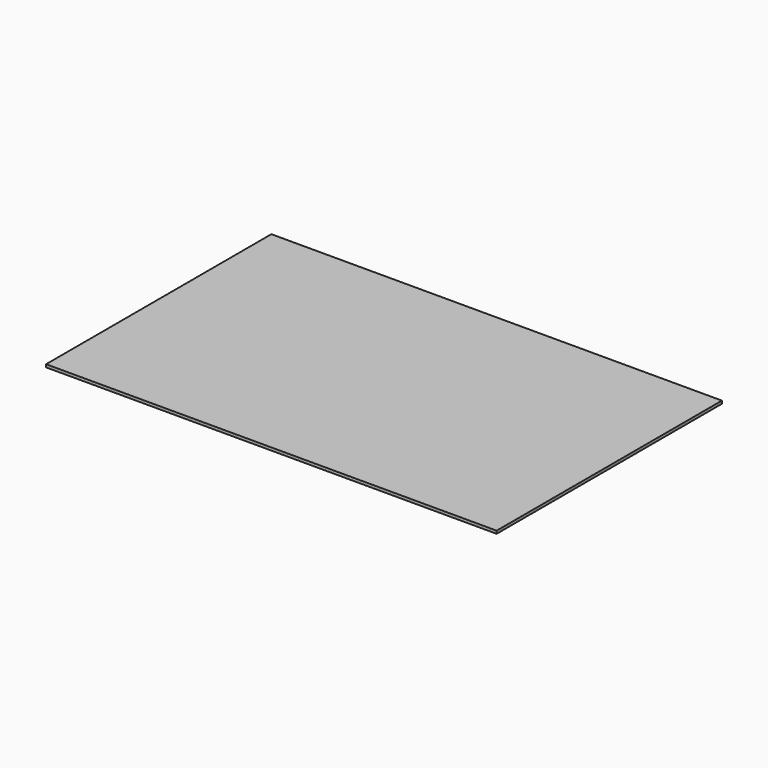
from build123d import *

# Parameters (mm, degrees)
F0_W     = 24384
F0_H     = 15240
F1_DEPTH = 152.4


# Not quite as in the source:
# - the program builds the solid bodies; features that only make, move or delete a surface that nothing else refers to are left out


with BuildPart() as f1:
    # F0 (on Top) → F1 (new body)
    with BuildSketch(Plane.XY):
        Rectangle(F0_W, F0_H)
    extrude(amount=F1_DEPTH)


solid = f1.part
